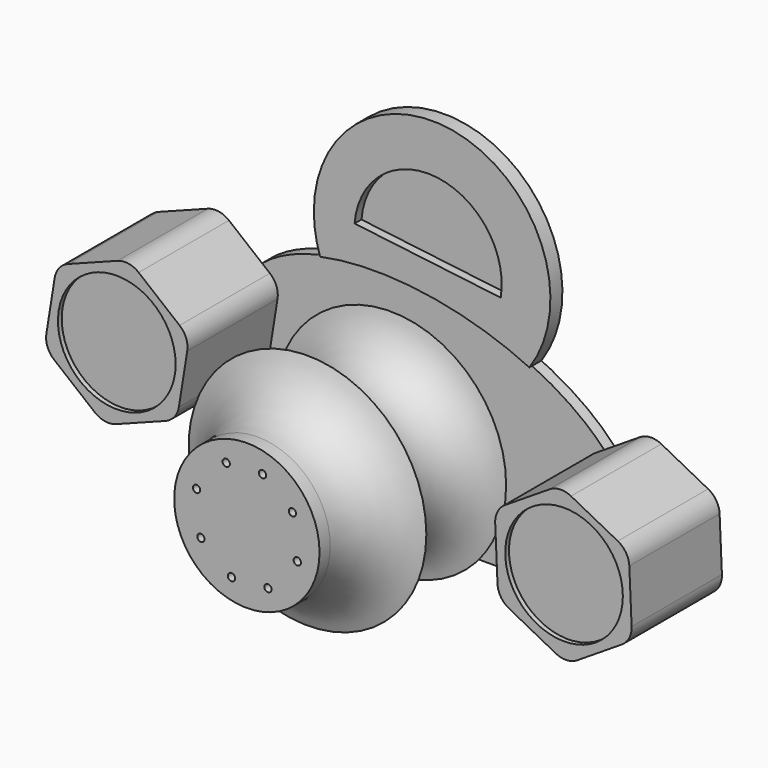
from build123d import *

# Parameters (mm, degrees)
F2_R         = 0.85
F3_DEPTH     = 16
F5_DEPTH     = 2.7
F7_DEPTH     = 25
F8_DEPTH     = 26.3
F9_DEPTH     = 25
F10_R        = 13.7081830223
F11_DEPTH    = 1.1
F12_T1_DEPTH = 26.3
F14_DEPTH    = 3.5
F16_DEPTH    = 6
F18_DEPTH    = 4.5


# Not quite as in the source:
# - a fillet or chamfer that OpenCascade refuses, or shapes differently, is made with other operations: its cross-section is extruded or revolved along the edge and cut away or added


with BuildPart() as f1:
    # F0 (on Top) → F1 (revolve)
    with BuildSketch(Plane.XY):
        with BuildLine():
            Line((0, 54.7616407275), (0, 0))
            Line((0, 0), (16.932335116, 0))
            Line((16.932335116, 0), (16.889732331, 3.1892883126))
            ThreePointArc((16.889732331, 3.1892883126), (19.8385918672, 12.257133335), (27.7038493693, 17.6478021561))
            ThreePointArc((27.7038493693, 17.6478021561), (16.4997519425, 29.4153527913), (26.8829930574, 41.9131666422))
            ThreePointArc((26.8829930574, 41.9131666422), (14.4092780208, 45.1495967178), (5.8257672936, 54.7616407275))
            Line((5.8257672936, 54.7616407275), (0, 54.7616407275))
        make_face()
    revolve(axis=Axis((0, 27.3808203638, 0), (0, 1, 0)))

    # F2 (on face) → F3 (cut)
    with BuildSketch(Plane.XZ):
        with Locations((-4.8139616118, 11.2955241897)):
            Circle(F2_R)
        with Locations((10.6174404705, 6.1670942083)):
            Circle(F2_R)
        with Locations((11.7574385329, -3.5391711268)):
            Circle(F2_R)
        with Locations((4.9072117267, -11.2553261254)):
            Circle(F2_R)
        with Locations((-10.7044627297, -6.0147793632)):
            Circle(F2_R)
        with Locations((-11.7096443523, 3.6942282364)):
            Circle(F2_R)
        with Locations((3.655111995, 11.7219132152)):
            Circle(F2_R)
        with Locations((-3.5784066248, -11.7455565704)):
            Circle(F2_R)
    extrude(amount=-F3_DEPTH, mode=Mode.SUBTRACT)


with BuildPart() as f5:
    # F4 (on face) → F5 (new body)
    with BuildSketch(Plane(origin=(0, 54.7616407275, 0), x_dir=(-1, 0, 0), z_dir=(0, 1, 0))):
        with BuildLine():
            add(Edge.make_bspline(
                [(-45.4141236842, -10.4606663808), (-35.9309916009, -51.6309052226), (27.4486278837, -15.3547862305), (90.8282473683, 20.9213327616), (17.9654958005, 25.8154526113), (-54.8972557674, 30.7095724609), (-45.4141236842, -10.4606663808)],
                knots=[0, 0, 0, 2.0943951024, 2.0943951024, 4.1887902048, 4.1887902048, 6.2831853072, 6.2831853072, 6.2831853072], degree=2, weights=[1, 0.5, 1, 0.5, 1, 0.5, 1]))
        make_face()
    extrude(amount=F5_DEPTH)

    # F6 (on face) → F7 (join)
    with BuildSketch(Plane.XZ.offset(-54.7616407275)):
        Polygon((51.7789917849, -23.1409610529), (67.008964544, -13.4359671261), (66.2191796394, 4.6060731456), (50.1994219757, 12.9431194905), (34.9694492166, 3.2381255638), (35.7592341212, -14.8039147079), align=None)
        Polygon((-55.9337141872, -9.1207021053), (-39.0623376148, -2.6789919353), (-36.2053339796, 15.1529038582), (-50.2197069168, 26.5430894817), (-67.0910834892, 20.1013793117), (-69.9480871244, 2.2694835183), align=None)
    extrude(amount=F7_DEPTH)

    # F6 (on face) → F8 (join)
    with BuildSketch(Plane.XZ.offset(-54.7616407275)):
        Polygon((51.7789917849, -23.1409610529), (67.008964544, -13.4359671261), (66.2191796394, 4.6060731456), (50.1994219757, 12.9431194905), (34.9694492166, 3.2381255638), (35.7592341212, -14.8039147079), align=None)
        Polygon((-55.9337141872, -9.1207021053), (-39.0623376148, -2.6789919353), (-36.2053339796, 15.1529038582), (-50.2197069168, 26.5430894817), (-67.0910834892, 20.1013793117), (-69.9480871244, 2.2694835183), align=None)
    extrude(amount=F8_DEPTH)

    # F6 (on face) → F9 (join)
    with BuildSketch(Plane.XZ.offset(-54.7616407275)):
        Polygon((51.7789917849, -23.1409610529), (67.008964544, -13.4359671261), (66.2191796394, 4.6060731456), (50.1994219757, 12.9431194905), (34.9694492166, 3.2381255638), (35.7592341212, -14.8039147079), align=None)
        Polygon((-55.9337141872, -9.1207021053), (-39.0623376148, -2.6789919353), (-36.2053339796, 15.1529038582), (-50.2197069168, 26.5430894817), (-67.0910834892, 20.1013793117), (-69.9480871244, 2.2694835183), align=None)
    extrude(amount=F9_DEPTH)

    # F10 (on face) → F11 (cut)
    with BuildSketch(Plane.XZ.offset(-28.4616407275)):
        with BuildLine():
            ThreePointArc((-39.3685275296, 8.7111936882), (-42.6449675564, 17.6046193413), (-50.9080612108, 22.2467484167))
            Line((-50.9080612108, 22.2467484167), (-53.076710552, 8.7111936882))
            Line((-53.076710552, 8.7111936882), (-39.5411558234, 6.5425443471))
            ThreePointArc((-39.5411558234, 6.5425443471), (-39.4117527529, 7.6234390637), (-39.3685275296, 8.7111936882))
        make_face()
        with BuildLine():
            Line((-53.076710552, 8.7111936882), (-50.9080612108, 22.2467484167))
            ThreePointArc((-50.9080612108, 22.2467484167), (-61.1143264325, 19.815742879), (-66.6122652805, 10.8798430294))
            Line((-66.6122652805, 10.8798430294), (-53.076710552, 8.7111936882))
        make_face()
        with BuildLine():
            Line((-39.5411558234, 6.5425443471), (-53.076710552, 8.7111936882))
            Line((-53.076710552, 8.7111936882), (-55.2453598931, -4.8243610403))
            ThreePointArc((-55.2453598931, -4.8243610403), (-45.0390946715, -2.3933555026), (-39.5411558234, 6.5425443471))
        make_face()
        with BuildLine():
            Line((-55.2453598931, -4.8243610403), (-53.076710552, 8.7111936882))
            Line((-53.076710552, 8.7111936882), (-66.6122652805, 10.8798430294))
            ThreePointArc((-66.6122652805, 10.8798430294), (-64.1812597428, 0.6735778077), (-55.2453598931, -4.8243610403))
        make_face()
        with Locations((51.1324964464, -5.002936814)):
            Circle(F10_R)
    extrude(amount=-F11_DEPTH, mode=Mode.SUBTRACT)

    # F12: fillet of radius 5 on 12 edges, made by hand

    # F12_s2 → F12_t1 (cut)
    with BuildSketch(Plane.XZ.offset(-54.7616407275)):
        with BuildLine():
            ThreePointArc((54.2134770538, -21.589634263), (51.7451643314, -22.3681983999), (49.2182607409, -21.8082983598))
            Line((49.2182607409, -21.8082983598), (49.172095951, -21.8970046852))
            Line((49.172095951, -21.8970046852), (51.7840416159, -23.2563206322))
            Line((51.7840416159, -23.2563206322), (54.2672165902, -21.6739673066))
            Line((54.2672165902, -21.6739673066), (54.2134770538, -21.589634263))
        make_face()
        with BuildLine():
            ThreePointArc((38.3199651652, -16.136577401), (36.411552483, -14.3882379474), (35.6329883461, -11.919925225))
            Line((35.6329883461, -11.919925225), (35.5330840199, -11.9242985069))
            Line((35.5330840199, -11.9242985069), (35.6618547105, -14.8659677795))
            Line((35.6618547105, -14.8659677795), (38.2738003754, -16.2252837265))
            Line((38.2738003754, -16.2252837265), (38.3199651652, -16.136577401))
        make_face()
        with BuildLine():
            ThreePointArc((66.8827187689, -10.5519776432), (66.3228187287, -13.0788812337), (64.5744792751, -14.9872939159))
            Line((64.5744792751, -14.9872939159), (64.6282188115, -15.0716269595))
            Line((64.6282188115, -15.0716269595), (67.1113937858, -13.4892736338))
            Line((67.1113937858, -13.4892736338), (66.9826230952, -10.5476043613))
            Line((66.9826230952, -10.5476043613), (66.8827187689, -10.5519776432))
        make_face()
        with BuildLine():
            ThreePointArc((63.6584485954, 5.9387358387), (65.5668612776, 4.190396385), (66.3454254145, 1.7220836627))
            Line((66.3454254145, 1.7220836627), (66.4453297408, 1.7264569446))
            Line((66.4453297408, 1.7264569446), (66.3165590502, 4.6681262172))
            Line((66.3165590502, 4.6681262172), (63.7046133853, 6.0274421641))
            Line((63.7046133853, 6.0274421641), (63.6584485954, 5.9387358387))
        make_face()
        with BuildLine():
            ThreePointArc((47.7649367068, 11.3917927007), (50.2332494292, 12.1703568376), (52.7601530198, 11.6104567974))
            Line((52.7601530198, 11.6104567974), (52.8063178096, 11.6991631229))
            Line((52.8063178096, 11.6991631229), (50.1943721447, 13.0584790698))
            Line((50.1943721447, 13.0584790698), (47.7111971705, 11.4761257442))
            Line((47.7111971705, 11.4761257442), (47.7649367068, 11.3917927007))
        make_face()
        with BuildLine():
            ThreePointArc((37.4039344856, 4.7894523536), (35.6555950319, 2.8810396714), (35.0956949918, 0.3541360809))
            Line((35.0956949918, 0.3541360809), (34.9957906655, 0.3497627989))
            Line((34.9957906655, 0.3497627989), (34.8670199749, 3.2914320715))
            Line((34.8670199749, 3.2914320715), (37.3501949492, 4.8737853971))
            Line((37.3501949492, 4.8737853971), (37.4039344856, 4.7894523536))
        make_face()
        with BuildLine():
            ThreePointArc((-53.2368533076, -8.0910056794), (-55.811345227, -8.3569401974), (-58.1738878899, -7.3000002859))
            Line((-58.1738878899, -7.3000002859), (-58.2369588511, -7.3776021794))
            Line((-58.2369588511, -7.3776021794), (-55.9519816743, -9.2347180351))
            Line((-55.9519816743, -9.2347180351), (-53.2011835771, -8.1844276807))
            Line((-53.2011835771, -8.1844276807), (-53.2368533076, -8.0910056794))
        make_face()
        with BuildLine():
            ThreePointArc((-69.4913999475, 5.1198817634), (-69.2254654296, 2.545389844), (-67.7079134216, 0.448781699))
            Line((-67.7079134216, 0.448781699), (-67.7709843828, 0.3711798055))
            Line((-67.7709843828, 0.3711798055), (-70.0559615596, 2.2282956612))
            Line((-70.0559615596, 2.2282956612), (-69.5901406391, 5.1357018713))
            Line((-69.5901406391, 5.1357018713), (-69.4913999475, 5.1198817634))
        make_face()
        with BuildLine():
            ThreePointArc((-38.6056504379, 0.1714063098), (-39.6625903494, -2.1911363532), (-41.7591984944, -3.7086883611))
            Line((-41.7591984944, -3.7086883611), (-41.7235287639, -3.8021103624))
            Line((-41.7235287639, -3.8021103624), (-38.9727306667, -2.7518200081))
            Line((-38.9727306667, -2.7518200081), (-38.5069097463, 0.1555862019))
            Line((-38.5069097463, 0.1555862019), (-38.6056504379, 0.1714063098))
        make_face()
        with BuildLine():
            ThreePointArc((-38.4455076823, 16.9736056775), (-36.9279556744, 14.8769975324), (-36.6620211565, 12.302505613))
            Line((-36.6620211565, 12.302505613), (-36.5632804648, 12.2866855052))
            Line((-36.5632804648, 12.2866855052), (-36.0974595444, 15.1940917152))
            Line((-36.0974595444, 15.1940917152), (-38.3824367212, 17.0512075709))
            Line((-38.3824367212, 17.0512075709), (-38.4455076823, 16.9736056775))
        make_face()
        with BuildLine():
            ThreePointArc((-47.979533214, 24.7223876624), (-50.342075877, 25.7793275738), (-52.9165677964, 25.5133930559))
            Line((-52.9165677964, 25.5133930559), (-52.9522375269, 25.6068150572))
            Line((-52.9522375269, 25.6068150572), (-50.2014394297, 26.6571054115))
            Line((-50.2014394297, 26.6571054115), (-47.9164622529, 24.7999895558))
            Line((-47.9164622529, 24.7999895558), (-47.979533214, 24.7223876624))
        make_face()
        with BuildLine():
            ThreePointArc((-67.547770666, 17.2509810666), (-66.4908307546, 19.6135237296), (-64.3942226095, 21.1310757376))
            Line((-64.3942226095, 21.1310757376), (-64.4298923401, 21.2244977389))
            Line((-64.4298923401, 21.2244977389), (-67.1806904373, 20.1742073845))
            Line((-67.1806904373, 20.1742073845), (-67.6465113577, 17.2668011745))
            Line((-67.6465113577, 17.2668011745), (-67.547770666, 17.2509810666))
        make_face()
    extrude(amount=F12_T1_DEPTH, mode=Mode.SUBTRACT)


with BuildPart() as f14:
    # F13 (on face) → F14 (new body)
    with BuildSketch(Plane(origin=(0, 57.4616407275, 0), x_dir=(-1, 0, 0), z_dir=(0, 1, 0))):
        with BuildLine():
            ThreePointArc((26.1125288837, 24.7082980765), (27.1963462363, 29.0575982583), (27.5608321849, 33.5250608623))
            ThreePointArc((27.5608321849, 33.5250608623), (-8.2113121209, 59.8342574289), (-22.6679721802, 17.8482465187))
            add(Edge.make_bspline(
                [(26.1125288837, 24.7082980765), (22.269737855, 25.5263408769), (17.9654958005, 25.8154526113), (-2.9314299342, 27.2190787005), (-22.6679721802, 17.8482465187)],
                knots=[3.9551466985, 3.9551466985, 3.9551466985, 4.1887902048, 4.1887902048, 5.1223774391, 5.1223774391, 5.1223774391], degree=2, weights=[0.9008883085, 0.9442217216, 1, 0.7771224653, 0.7529425125]))
        make_face()
    extrude(amount=-F14_DEPTH)

    # F15 (on face) → F16 (join)
    with BuildSketch(Plane(origin=(0, 57.4616407275, 0), x_dir=(-1, 0, 0), z_dir=(0, 1, 0))):
        with BuildLine():
            Line((-15.9830935299, 29.9917142838), (18.0653184652, 34.1367051005))
            ThreePointArc((18.0653184652, 34.1367051005), (-1.0872723755, 49.5475111585), (-15.9830935299, 29.9917142838))
        make_face()
    extrude(amount=-F16_DEPTH)

    # F17 (on face) → F18 (cut)
    with BuildSketch(Plane.XZ.offset(-51.4616407275)):
        with BuildLine():
            Line((-18.0653184652, 34.1367051005), (15.9830935299, 29.9917142838))
            ThreePointArc((15.9830935299, 29.9917142838), (1.1221978062, 49.8344009265), (-18.0653184652, 34.1367051005))
        make_face()
    extrude(amount=-F18_DEPTH, mode=Mode.SUBTRACT)


solid = Compound([f1.part, f5.part, f14.part])
